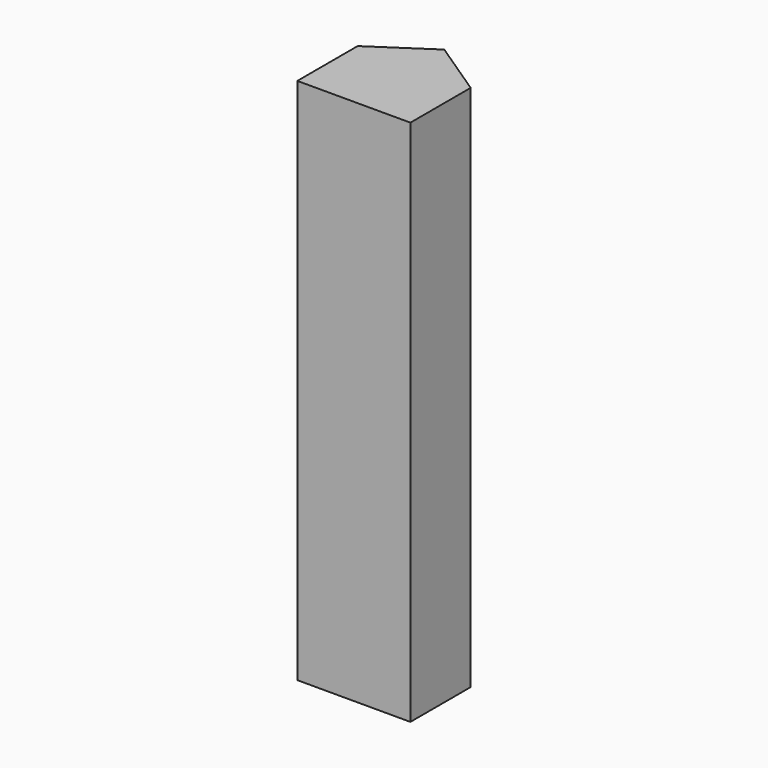
from build123d import *

# Parameters (mm, degrees)
F1_DEPTH       = 711.2
F3_D           = 5.5
F3_DEPTH       = 25.4
F3_CBORE_D     = 9.75
F3_CBORE_DEPTH = 5
F3_TIP         = 1.6523667023


# Not quite as in the source:
# - a feature names something its author has since deleted; it is built from what else it names


with BuildPart() as f1:
    # F0 (on Top) → F1 (new body)
    with BuildSketch(Plane.XY):
        Polygon((0, 101.6), (0, 0), (152.4, 0), (152.4, 101.6), (76.2, 152.4), align=None)
    extrude(amount=F1_DEPTH)

    # F3
    with Locations(Plane(origin=(0, 0, 0), x_dir=(1, 0, 0), z_dir=(0, 0, -1))):
        with Locations((100.9017452598, -60.0949265063), (67.4944594502, -83.0287188292)):
            CounterBoreHole(F3_D / 2, F3_CBORE_D / 2, F3_CBORE_DEPTH, depth=F3_DEPTH)
            with Locations((0, 0, -(F3_DEPTH + F3_TIP / 2))):  # 118° drill point
                Cone(0, F3_D / 2, F3_TIP, mode=Mode.SUBTRACT)


solid = f1.part
